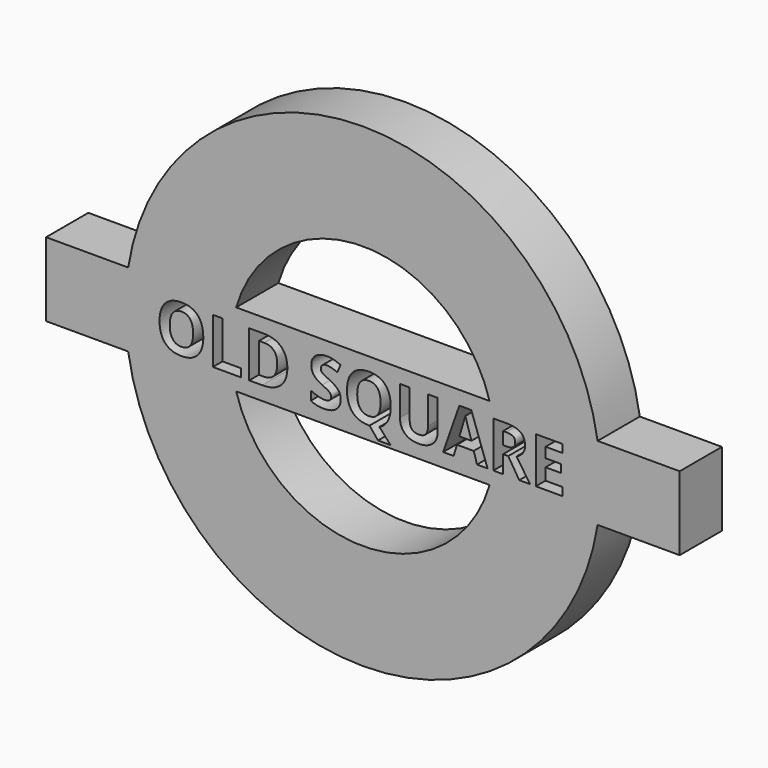
from build123d import *

# Parameters (mm, degrees)
F0_R         = 2.25
F0_R_2       = 1.25
F1_DEPTH     = 0.5
F2_W         = 6
F2_H         = 0.7
F3_DEPTH     = 0.5
F4_TEXT_SIZE = 0.6095200661
F5_DEPTH     = 0.5


# Not quite as in the source:
# - Text() gives the source's letters only with a copy of the font that has no kerning and outlines rounded to 1/6400 em; it was checked with that copy


with BuildPart() as f1:
    # F0 (on Front) → F1 (new body)
    with BuildSketch(Plane.XZ):
        Circle(F0_R)
        Circle(F0_R_2, mode=Mode.SUBTRACT)
    extrude(amount=F1_DEPTH)

    # F2 (on Front) → F3 (join)
    with BuildSketch(Plane.XZ):
        Rectangle(F2_W, F2_H)
    extrude(amount=F3_DEPTH)

    # F4 (on Front) → F5 (cut, through all)
    with BuildSketch(Plane.XZ):
        with Locations((-1.960742753, -0.218488276)):
            Text('OLD SQUARE', F4_TEXT_SIZE, font='Open Sans', font_style=FontStyle.BOLD, text_align=(TextAlign.LEFT, TextAlign.BOTTOM))
    extrude(amount=F5_DEPTH, mode=Mode.SUBTRACT)


solid = f1.part
